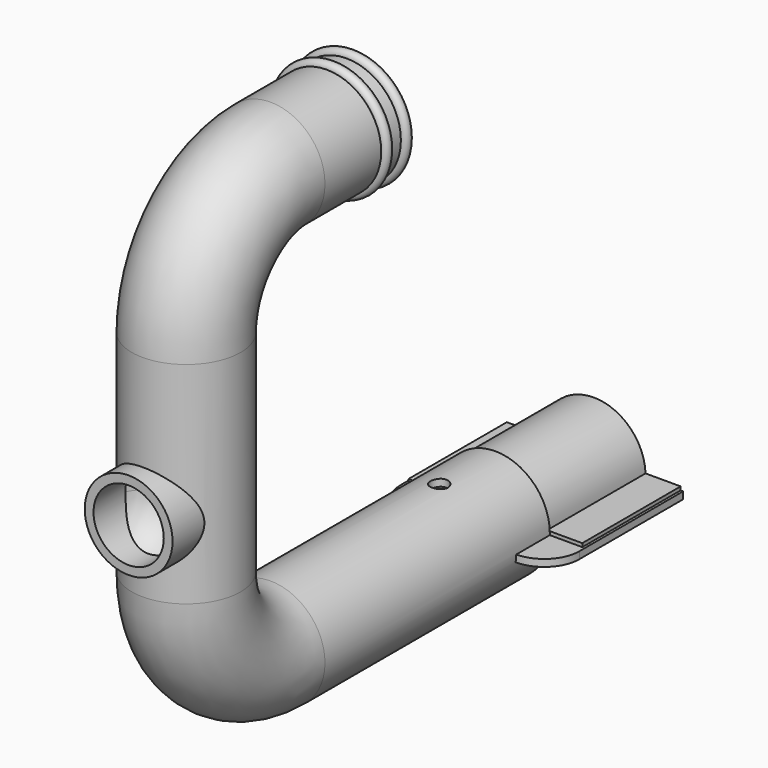
from build123d import *

# Parameters (mm, degrees)
F0_R      = 14.15
F1_DEPTH  = 17.5
F3_R      = 15.5
F3_R_2    = 13.5
F11_R     = 2.5
F12_DEPTH = 137.0010001
F18_DEPTH = 2
F23_DEPTH = 30
F26_ANGLE = 90
F27_W     = 6.0253508091
F27_H     = 56.4770405108
F20_R     = 12.5
F30_R     = 10
F31_DEPTH = 11.4318215269


with BuildPart() as f1:
    # F0 (on Front) → F1 (new body, symmetric)
    with BuildSketch(Plane.XZ):
        with BuildLine():
            Line((24.7415229878, 0.5), (14.7415229878, 0.5))
            ThreePointArc((14.7415229878, 0.5), (0, 14.75), (-14.7415229878, 0.5))
            Line((-14.7415229878, 0.5), (-24.7415229878, 0.5))
            Line((-24.7415229878, 0.5), (-24.7415229878, -0.5))
            Line((-24.7415229878, -0.5), (-14.7415229878, -0.5))
            ThreePointArc((-14.7415229878, -0.5), (0, -14.75), (14.7415229878, -0.5))
            Line((14.7415229878, -0.5), (24.7415229878, -0.5))
            Line((24.7415229878, -0.5), (24.7415229878, 0.5))
        make_face()
        Circle(F0_R, mode=Mode.SUBTRACT)
    extrude(amount=F1_DEPTH, both=True)


with BuildPart() as f4:
    # F4: sweep along a path in F2
    with BuildLine(Plane.YZ) as f4_path:
        Line((-17.5, 0), (-97.5, 0))
        ThreePointArc((-97.5, 0), (-118.7132034356, 8.7867965644), (-127.5, 30))
        Line((-127.5, 30), (-127.5, 90))
        ThreePointArc((-127.5, 90), (-118.7132034356, 111.2132034356), (-97.5, 120))
        Line((-97.5, 120), (-67.5, 120))
    # F3 (on face) → F4 (sweep)
    with BuildSketch(Plane.XZ.offset(17.5)):
        Circle(F3_R)
        Circle(F3_R_2, mode=Mode.SUBTRACT)
    sweep(path=f4_path.line)

    # F9 (on Right) → F10 (revolve)
    with BuildSketch(Plane.YZ):
        with BuildLine():
            Line((-70.5, 135.5), (-67.5, 135.5))
            ThreePointArc((-67.5, 135.5), (-69, 137), (-70.5, 135.5))
        make_face()
        with BuildLine():
            Line((-77.5, 135.5), (-74.5, 135.5))
            ThreePointArc((-74.5, 135.5), (-76, 137), (-77.5, 135.5))
        make_face()
    revolve(axis=Axis((0, -82.5, 120), (0, 1, 0)))

    # F11 (on Top) → F12 (cut, through all)
    with BuildSketch(Plane.XY):
        with Locations((0, -37.5)):
            Circle(F11_R)
    extrude(amount=F12_DEPTH, mode=Mode.SUBTRACT)

    # F17 (on offset) → F18 (join)
    with BuildSketch(Plane(origin=(0, 0, -0.5), x_dir=(1, 0, 0), z_dir=(0, 0, -1))):
        with BuildLine():
            Line((-25.4652393452, 19.4262243624), (-25.4652393452, -17.5))
            Line((-25.4652393452, -17.5), (-14.846339575, -17.5))
            Line((-14.846339575, -17.5), (-14.846339575, 17.5))
            Line((-14.846339575, 17.5), (-14.5169012249, 17.5))
            Line((-14.5169012249, 17.5), (-14.5169012249, 29.4262243624))
            Line((-14.5169012249, 29.4262243624), (-14.846339575, 29.4262243624))
            Line((-14.846339575, 29.4262243624), (-15.4652393452, 29.4262243624))
            ThreePointArc((-15.4652393452, 29.4262243624), (-22.5363071571, 26.4972921743), (-25.4652393452, 19.4262243624))
        make_face()
        with BuildLine():
            Line((14.5169012249, 29.4262243624), (14.5169012249, 17.5))
            Line((14.5169012249, 17.5), (14.846339575, 17.5))
            Line((14.846339575, 17.5), (14.846339575, -17.5))
            Line((14.846339575, -17.5), (25.4652393452, -17.5))
            Line((25.4652393452, -17.5), (25.4652393452, 19.4262243624))
            ThreePointArc((25.4652393452, 19.4262243624), (22.5363071571, 26.4972921743), (15.4652393452, 29.4262243624))
            Line((15.4652393452, 29.4262243624), (14.846339575, 29.4262243624))
            Line((14.846339575, 29.4262243624), (14.5169012249, 29.4262243624))
        make_face()
    extrude(amount=F18_DEPTH)

    # F19 (on offset) → F23 (join, through all)
    with BuildSketch(Plane.XY.offset(80)):
        with BuildLine():
            ThreePointArc((10.5790063475, -135.8865740741), (11.165200766, -135.0886950034), (11.6913429511, -134.25))
            ThreePointArc((11.6913429511, -134.25), (0, -127.5), (-11.6913429511, -134.25))
            ThreePointArc((-11.6913429511, -134.25), (-11.165200766, -135.0886950034), (-10.5790063475, -135.8865740741))
            ThreePointArc((-10.5790063475, -135.8865740741), (0, -129.25), (10.5790063475, -135.8865740741))
        make_face()
    extrude(amount=-F23_DEPTH)

    # F25 (on plane+point) → F26 (revolve)
    with BuildSketch(Plane.XY.offset(50)):
        with BuildLine():
            ThreePointArc((10.5790063475, -135.8865740741), (11.165200766, -135.0886950034), (11.6913429511, -134.25))
            ThreePointArc((11.6913429511, -134.25), (0, -127.5), (-11.6913429511, -134.25))
            ThreePointArc((-11.6913429511, -134.25), (-11.165200766, -135.0886950034), (-10.5790063475, -135.8865740741))
            ThreePointArc((-10.5790063475, -135.8865740741), (0, -129.25), (10.5790063475, -135.8865740741))
        make_face()
    revolve(axis=Axis((0.5745105445, -143, 50), (-1, 0, 0)), revolution_arc=F26_ANGLE)

    # F27 (on Right) → F28 (revolve, cut)
    with BuildSketch(Plane.YZ):
        with Locations((-146.0126754045, 61.7614797446)):
            Rectangle(F27_W, F27_H)
    revolve(axis=Axis((0, -127.5, 60), (0, 0, 1)), mode=Mode.SUBTRACT)

    # F20 (on offset) → F29 (join, up to the next surface of F4)
    with BuildSketch(Plane.XZ.offset(148)):
        with Locations((0, 50)):
            Circle(F20_R)
    extrude(until=Until.NEXT, dir=(0, 1, 0))

    # F30 (on face) → F31 (cut, through all)
    with BuildSketch(Plane.XZ.offset(148)):
        with Locations((0, 50)):
            Circle(F30_R)
    extrude(amount=-F31_DEPTH, mode=Mode.SUBTRACT)


solid = Compound([f1.part, f4.part])
